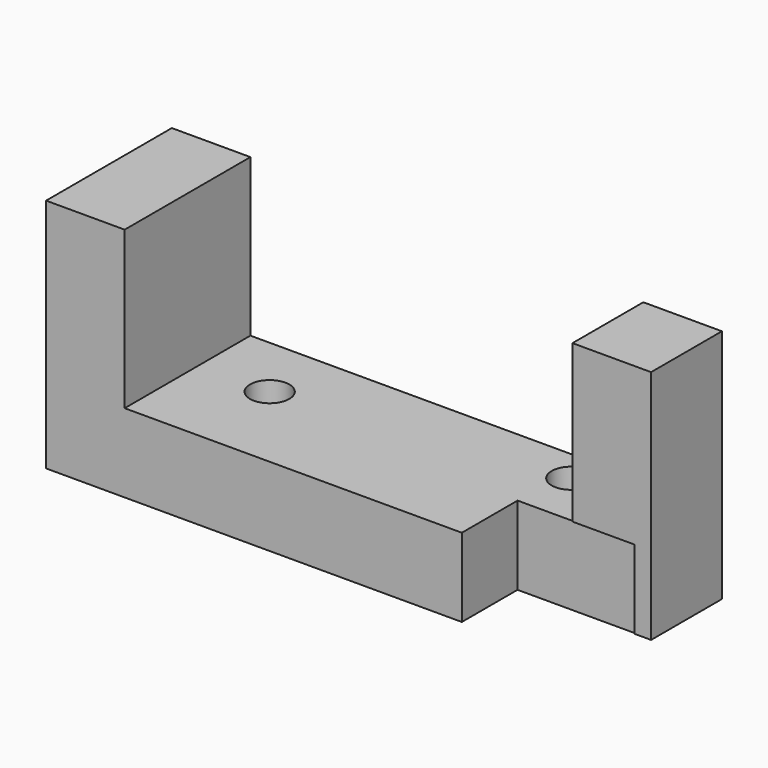
from build123d import *

# Parameters (mm, degrees)
F0_W      = 88.9
F0_H      = 50.8
F1_DEPTH  = 25.4
F2_W      = 63.5
F2_H      = 25.4
F3_DEPTH  = 25.401
F4_W      = 88.9
F4_H      = 12.7
F5_DEPTH  = 25.401
F8_W      = 19.05
F8_H      = 11.447972618
F9_DEPTH  = 12.701
F10_W     = 12.7
F10_H     = 11.090603964
F11_DEPTH = 38.101
F12_R     = 3.175
F14_DEPTH = 12.701
F13_R     = 3.175
F15_DEPTH = 12.701


# Not quite as in the source:
# - a feature of the source that left no trace in its solid (it failed there, or was rolled back) is left out


with BuildPart() as f1:
    # F0 (on Front) → F1 (new body)
    with BuildSketch(Plane.XZ):
        Rectangle(F0_W, F0_H)
    extrude(amount=F1_DEPTH)

    # F2 (on face) → F3 (cut, through all)
    with BuildSketch(Plane.XZ.offset(25.4)):
        with Locations((0, 12.7)):
            Rectangle(F2_W, F2_H)
    extrude(amount=-F3_DEPTH, mode=Mode.SUBTRACT)

    # F4 (on face) → F5 (cut, through all)
    with BuildSketch(Plane.XZ.offset(25.4)):
        with Locations((0, -19.05)):
            Rectangle(F4_W, F4_H)
    extrude(amount=-F5_DEPTH, mode=Mode.SUBTRACT)

    # F8 (on face) → F9 (cut, through all)
    with BuildSketch(Plane.XY):
        with Locations((32.2608303964, -19.8649899103)):
            Rectangle(F8_W, F8_H)
    extrude(amount=-F9_DEPTH, mode=Mode.SUBTRACT)

    # F10 (on face) → F11 (cut, through all)
    with BuildSketch(Plane.XY.offset(25.4)):
        with Locations((38.1, -19.854698018)):
            Rectangle(F10_W, F10_H)
    extrude(amount=-F11_DEPTH, mode=Mode.SUBTRACT)

    # F12 (on face) → F14 (cut, through all)
    with BuildSketch(Plane.XY):
        with Locations((24.2214165628, -5.1358360797)):
            Circle(F12_R)
    extrude(amount=-F14_DEPTH, mode=Mode.SUBTRACT)

    # F13 (on face) → F15 (cut, through all)
    with BuildSketch(Plane.XY):
        with Locations((-20.2783960849, -10.4468446225)):
            Circle(F13_R)
    extrude(amount=-F15_DEPTH, mode=Mode.SUBTRACT)


solid = f1.part
